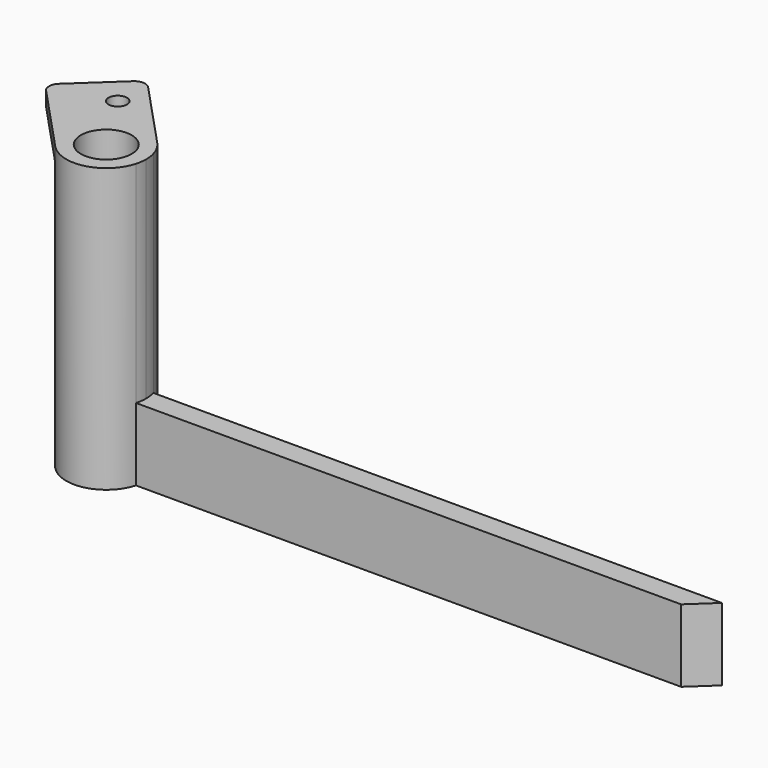
from build123d import *

# Parameters (mm, degrees)
F1_DEPTH = 10
F2_DEPTH = 39
F3_R     = 1.27
F4_DEPTH = 39
F0_R     = 1.27
F5_DEPTH = 37


# Not quite as in the source:
# - a feature names something its author has since deleted; it is built from what else it names


with BuildPart() as f1:
    # F0 (on Top) → F1 (new body)
    with BuildSketch(Plane.XY):
        with BuildLine():
            Line((39.0916730868, 1.5), (-39.2084973779, 1.5))
            ThreePointArc((-39.2084973779, 1.5), (-39.0523737086, 0.7572105316), (-39, 0))
            ThreePointArc((-39, 0), (-39.0523737086, -0.7572105316), (-39.2084973779, -1.5))
            Line((-39.2084973779, -1.5), (35.8745669567, -1.5))
            Line((35.8745669567, -1.5), (39.0916730868, 1.5))
        make_face()
    extrude(amount=F1_DEPTH)

    # F0 (on Top) → F2 (join)
    with BuildSketch(Plane.XY):
        with BuildLine():
            ThreePointArc((-47.0597379557, -2.3869942602), (-46.8869942602, 2.5597379557), (-41.9402620443, 2.3869942602))
            Line((-41.9402620443, 2.3869942602), (-40.4775546411, 3.7509909803))
            ThreePointArc((-40.4775546411, 3.7509909803), (-48.2509909803, 4.0224453589), (-48.5224453589, -3.7509909803))
            Line((-48.5224453589, -3.7509909803), (-47.0597379557, -2.3869942602))
        make_face()
        with BuildLine():
            ThreePointArc((-41.9402620443, 2.3869942602), (-41.2435385121, 1.2827542935), (-41, 0))
            ThreePointArc((-41, 0), (-43.2172457065, -3.2564614879), (-47.0597379557, -2.3869942602))
            Line((-47.0597379557, -2.3869942602), (-48.5224453589, -3.7509909803))
            ThreePointArc((-48.5224453589, -3.7509909803), (-43.2079602627, -5.346085794), (-39.2084973779, -1.5))
            ThreePointArc((-39.2084973779, -1.5), (-39.0523737086, -0.7572105316), (-39, 0))
            ThreePointArc((-39, 0), (-39.0523737086, 0.7572105316), (-39.2084973779, 1.5))
            ThreePointArc((-39.2084973779, 1.5), (-39.7089513834, 2.7010836998), (-40.4775546411, 3.7509909803))
            Line((-40.4775546411, 3.7509909803), (-41.9402620443, 2.3869942602))
        make_face()
    extrude(amount=F2_DEPTH)

    # F3 (on face) → F4 (join)
    with BuildSketch(Plane.XY):
        with BuildLine():
            Line((-57.3884240397, 5.7566071407), (-48.5224453589, -3.7509909803))
            ThreePointArc((-48.5224453589, -3.7509909803), (-48.2509909803, 4.0224453589), (-40.4775546411, 3.7509909803))
            Line((-40.4775546411, 3.7509909803), (-49.3435333219, 13.2585891014))
            ThreePointArc((-49.3435333219, 13.2585891014), (-50.3882146293, 13.7346778018), (-51.4635614144, 13.3326221137))
            Line((-51.4635614144, 13.3326221137), (-57.3143910274, 7.8766352332))
            ThreePointArc((-57.3143910274, 7.8766352332), (-57.7904797278, 6.8319539259), (-57.3884240397, 5.7566071407))
        make_face()
        with Locations((-49.8572761974, 8.6775337363)):
            Circle(F3_R, mode=Mode.SUBTRACT)
    extrude(amount=F4_DEPTH)

    # F0 (on Top) → F5 (cut)
    with BuildSketch(Plane.XY):
        with BuildLine():
            ThreePointArc((-48.5224453589, -3.7509909803), (-48.2509909803, 4.0224453589), (-40.4775546411, 3.7509909803))
            Line((-40.4775546411, 3.7509909803), (-49.3435333219, 13.2585891014))
            ThreePointArc((-49.3435333219, 13.2585891014), (-50.3882146293, 13.7346778018), (-51.4635614144, 13.3326221137))
            Line((-51.4635614144, 13.3326221137), (-57.3143910274, 7.8766352332))
            ThreePointArc((-57.3143910274, 7.8766352332), (-57.7904797278, 6.8319539259), (-57.3884240397, 5.7566071407))
            Line((-57.3884240397, 5.7566071407), (-48.5224453589, -3.7509909803))
        make_face()
        with Locations((-49.8572761974, 8.6775337363)):
            Circle(F0_R, mode=Mode.SUBTRACT)
    extrude(amount=F5_DEPTH, mode=Mode.SUBTRACT)


solid = f1.part
